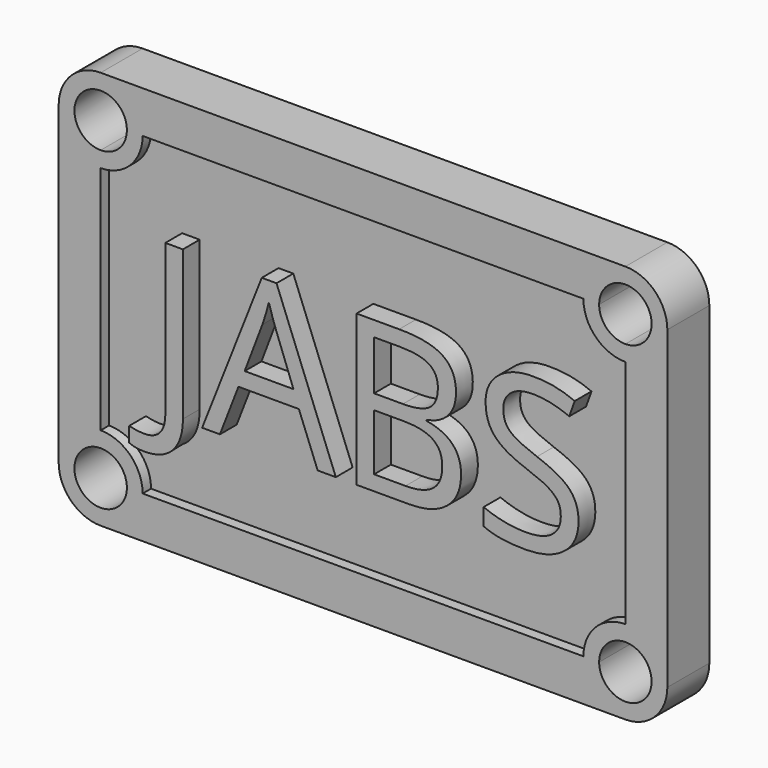
from build123d import *

# Parameters (mm, degrees)
F1_DEPTH     = 6.35
F2_DEPTH     = 5.08
F3_DEPTH     = 25.4
F4_TEXT_SIZE = 25.5638073819
F5_DEPTH     = 2.54


# Not quite as in the source:
# - Text() gives the source's letters only with a copy of the font that has no kerning and outlines rounded to 1/6400 em; it was checked with that copy


with BuildPart() as f1:
    # F0 (on Front) → F1 (new body)
    with BuildSketch(Plane.XZ):
        with BuildLine():
            ThreePointArc((68.58, 0), (67.0921024484, -3.5921024484), (63.5, -5.08))
            Line((63.5, -5.08), (63.5, -33.02))
            ThreePointArc((63.5, -33.02), (67.0921024484, -34.5078975516), (68.58, -38.1))
            Line((68.58, -38.1), (68.58, 0))
        make_face()
        with BuildLine():
            ThreePointArc((0, 5.08), (3.5921024484, 3.5921024484), (5.08, 0))
            Line((5.08, 0), (58.42, 0))
            ThreePointArc((58.42, 0), (59.9078975516, 3.5921024484), (63.5, 5.08))
            Line((63.5, 5.08), (0, 5.08))
        make_face()
        with BuildLine():
            Line((0, -33.02), (0, -5.08))
            ThreePointArc((0, -5.08), (-3.5921024484, -3.5921024484), (-5.08, 0))
            Line((-5.08, 0), (-5.08, -38.1))
            ThreePointArc((-5.08, -38.1), (-3.5921024484, -34.5078975516), (0, -33.02))
        make_face()
        with BuildLine():
            Line((58.42, -38.1), (5.08, -38.1))
            ThreePointArc((5.08, -38.1), (3.5921024484, -41.6921024484), (0, -43.18))
            Line((0, -43.18), (63.5, -43.18))
            ThreePointArc((63.5, -43.18), (59.9078975516, -41.6921024484), (58.42, -38.1))
        make_face()
        with BuildLine():
            ThreePointArc((63.5, 5.08), (59.9078975516, 3.5921024484), (58.42, 0))
            Line((58.42, 0), (60.325, 0))
            ThreePointArc((60.325, 0), (63.5, 3.175), (66.675, 0))
            ThreePointArc((66.675, 0), (65.7450640303, -2.2450640303), (63.5, -3.175))
            Line((63.5, -3.175), (63.5, -5.08))
            ThreePointArc((63.5, -5.08), (67.0921024484, -3.5921024484), (68.58, 0))
            ThreePointArc((68.58, 0), (67.0921024484, 3.5921024484), (63.5, 5.08))
        make_face()
        with BuildLine():
            Line((60.325, 0), (58.42, 0))
            ThreePointArc((58.42, 0), (59.9078975516, -3.5921024484), (63.5, -5.08))
            Line((63.5, -5.08), (63.5, -3.175))
            ThreePointArc((63.5, -3.175), (61.2549359697, -2.2450640303), (60.325, 0))
        make_face()
        with BuildLine():
            ThreePointArc((68.58, -38.1), (67.0921024484, -34.5078975516), (63.5, -33.02))
            Line((63.5, -33.02), (63.5, -34.925))
            ThreePointArc((63.5, -34.925), (65.7450640303, -35.8549359697), (66.675, -38.1))
            ThreePointArc((66.675, -38.1), (63.5, -41.275), (60.325, -38.1))
            Line((60.325, -38.1), (58.42, -38.1))
            ThreePointArc((58.42, -38.1), (59.9078975516, -41.6921024484), (63.5, -43.18))
            ThreePointArc((63.5, -43.18), (67.0921024484, -41.6921024484), (68.58, -38.1))
        make_face()
        with BuildLine():
            Line((63.5, -34.925), (63.5, -33.02))
            ThreePointArc((63.5, -33.02), (59.9078975516, -34.5078975516), (58.42, -38.1))
            Line((58.42, -38.1), (60.325, -38.1))
            ThreePointArc((60.325, -38.1), (61.2549359697, -35.8549359697), (63.5, -34.925))
        make_face()
        with BuildLine():
            Line((0, -34.925), (0, -33.02))
            ThreePointArc((0, -33.02), (-3.5921024484, -34.5078975516), (-5.08, -38.1))
            ThreePointArc((-5.08, -38.1), (-3.5921024484, -41.6921024484), (0, -43.18))
            ThreePointArc((0, -43.18), (3.5921024484, -41.6921024484), (5.08, -38.1))
            Line((5.08, -38.1), (3.175, -38.1))
            ThreePointArc((3.175, -38.1), (-2.2450640303, -40.3450640303), (0, -34.925))
        make_face()
        with BuildLine():
            ThreePointArc((5.08, -38.1), (3.5921024484, -34.5078975516), (0, -33.02))
            Line((0, -33.02), (0, -34.925))
            ThreePointArc((0, -34.925), (2.2450640303, -35.8549359697), (3.175, -38.1))
            Line((3.175, -38.1), (5.08, -38.1))
        make_face()
        with BuildLine():
            Line((5.08, 0), (3.175, 0))
            ThreePointArc((3.175, 0), (2.2450640303, -2.2450640303), (0, -3.175))
            Line((0, -3.175), (0, -5.08))
            ThreePointArc((0, -5.08), (3.5921024484, -3.5921024484), (5.08, 0))
        make_face()
        with BuildLine():
            ThreePointArc((0, -3.175), (-2.2450640303, 2.2450640303), (3.175, 0))
            Line((3.175, 0), (5.08, 0))
            ThreePointArc((5.08, 0), (3.5921024484, 3.5921024484), (0, 5.08))
            ThreePointArc((0, 5.08), (-3.5921024484, 3.5921024484), (-5.08, 0))
            ThreePointArc((-5.08, 0), (-3.5921024484, -3.5921024484), (0, -5.08))
            Line((0, -5.08), (0, -3.175))
        make_face()
    extrude(amount=F1_DEPTH)

    # F0 (on Front) → F2 (join)
    with BuildSketch(Plane.XZ):
        with BuildLine():
            Line((58.42, 0), (5.08, 0))
            ThreePointArc((5.08, 0), (3.5921024484, -3.5921024484), (0, -5.08))
            Line((0, -5.08), (0, -33.02))
            ThreePointArc((0, -33.02), (3.5921024484, -34.5078975516), (5.08, -38.1))
            Line((5.08, -38.1), (58.42, -38.1))
            ThreePointArc((58.42, -38.1), (59.9078975516, -34.5078975516), (63.5, -33.02))
            Line((63.5, -33.02), (63.5, -5.08))
            ThreePointArc((63.5, -5.08), (59.9078975516, -3.5921024484), (58.42, 0))
        make_face()
    extrude(amount=F2_DEPTH)

    # F0 (on Front) → F3 (cut)
    with BuildSketch(Plane.XZ):
        with BuildLine():
            Line((3.175, 0), (0, 0))
            Line((0, 0), (0, -3.175))
            ThreePointArc((0, -3.175), (2.2450640303, -2.2450640303), (3.175, 0))
        make_face()
    extrude(amount=-F3_DEPTH, mode=Mode.SUBTRACT)


with BuildPart() as f5:
    # F4 (on face) → F5 (new body)
    with BuildSketch(Plane.XZ.offset(5.08)):
        with Locations((10.0279524922, -31.2094651163)):
            Text('JABS', F4_TEXT_SIZE, font='Open Sans', text_align=(TextAlign.LEFT, TextAlign.BOTTOM))
    extrude(amount=F5_DEPTH)


with BuildPart() as f5_1:
    # F6: moved
    add(f5.part.moved(Location((-5.08, 0, 3.302))))


with BuildPart() as f5_2:
    # F7: moved
    add(f5_1.part.moved(Location((1.524, 0, 0))))


solid = Compound([f1.part, f5_2.part])
